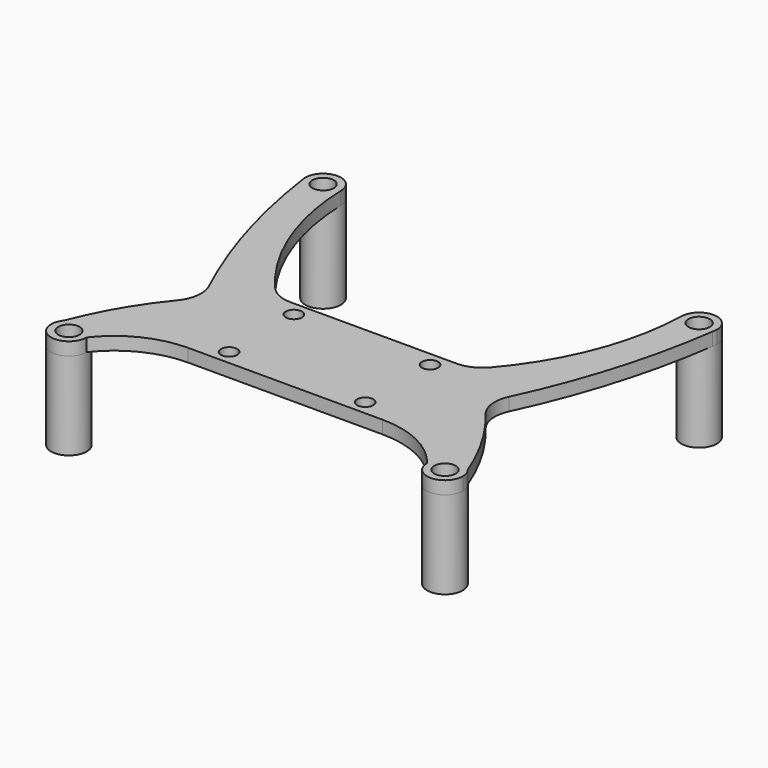
from build123d import *

# Parameters (mm, degrees)
F0_W     = 30
F0_H     = 17
F1_DEPTH = 2
F2_R     = 2.75
F3_DEPTH = 13.5
F4_R     = 5
F5_D     = 3.3
F5_DEPTH = 13.501
F6_D     = 3.3
F7_D     = 2.5


with BuildPart() as f1:
    # F0 (on Top) → F1 (new body)
    with BuildSketch(Plane.XY):
        with BuildLine():
            ThreePointArc((-31.125909, 1.744423), (-31.446933, 0.875424), (-31.75, 0))
            ThreePointArc((-31.75, 0), (-29, -2.75), (-26.25, 0))
            ThreePointArc((-26.25, 0), (-28.073649, 2.589281), (-31.125909, 1.744423))
        make_face()
        with BuildLine():
            ThreePointArc((-31.125909, 1.744423), (-31.589281, 0.926351), (-31.75, 0))
            ThreePointArc((-31.75, 0), (-31.446933, 0.875424), (-31.125909, 1.744423))
        make_face()
        with BuildLine():
            ThreePointArc((-31.125909, 1.744423), (-28.073649, 2.589281), (-26.25, 0))
            ThreePointArc((-26.25, 0), (-21.26124, 4.0514), (-15, 5.5))
            ThreePointArc((-15, 5.5), (-18.527929, 11.002842), (-21.688812, 16.724413))
            ThreePointArc((-21.688812, 16.724413), (-27.151344, 9.703113), (-31.125909, 1.744423))
        make_face()
        with Locations((0, 14)):
            Rectangle(F0_W, F0_H)
        with BuildLine():
            ThreePointArc((-21.688812, 16.724413), (-18.527929, 11.002842), (-15, 5.5))
            Line((-15, 5.5), (-15, 22.5))
            ThreePointArc((-15, 22.5), (-18.486529, 19.776801), (-21.688812, 16.724413))
        make_face()
        with BuildLine():
            ThreePointArc((-31.648811, 48.26088), (-27.981561, 32.078047), (-21.688812, 16.724413))
            ThreePointArc((-21.688812, 16.724413), (-18.486529, 19.776801), (-15, 22.5))
            ThreePointArc((-15, 22.5), (-23.091727, 34.702805), (-26.25, 49))
            ThreePointArc((-26.25, 49), (-28.626993, 46.275415), (-31.648811, 48.26088))
        make_face()
        with BuildLine():
            ThreePointArc((21.688812, 16.724413), (18.527929, 11.002842), (15, 5.5))
            ThreePointArc((15, 5.5), (21.26124, 4.0514), (26.25, 0))
            ThreePointArc((26.25, 0), (28.073649, 2.589281), (31.125909, 1.744423))
            ThreePointArc((31.125909, 1.744423), (27.151344, 9.703113), (21.688812, 16.724413))
        make_face()
        with BuildLine():
            Line((15, 22.5), (15, 5.5))
            ThreePointArc((15, 5.5), (18.527929, 11.002842), (21.688812, 16.724413))
            ThreePointArc((21.688812, 16.724413), (18.486529, 19.776801), (15, 22.5))
        make_face()
        with BuildLine():
            ThreePointArc((-31.75, 49), (-31.700095, 48.630345), (-31.648811, 48.26088))
            ThreePointArc((-31.648811, 48.26088), (-28.626993, 46.275415), (-26.25, 49))
            ThreePointArc((-26.25, 49), (-29, 51.75), (-31.75, 49))
        make_face()
        with BuildLine():
            ThreePointArc((-31.75, 49), (-31.724585, 48.626993), (-31.648811, 48.26088))
            ThreePointArc((-31.648811, 48.26088), (-31.700095, 48.630345), (-31.75, 49))
        make_face()
        with BuildLine():
            ThreePointArc((26.25, 49), (23.091727, 34.702805), (15, 22.5))
            ThreePointArc((15, 22.5), (18.486529, 19.776801), (21.688812, 16.724413))
            ThreePointArc((21.688812, 16.724413), (27.981561, 32.078047), (31.648811, 48.26088))
            ThreePointArc((31.648811, 48.26088), (28.626993, 46.275415), (26.25, 49))
        make_face()
        with BuildLine():
            ThreePointArc((31.125909, 1.744423), (28.073649, 2.589281), (26.25, 0))
            ThreePointArc((26.25, 0), (29, -2.75), (31.75, 0))
            ThreePointArc((31.75, 0), (31.446933, 0.875424), (31.125909, 1.744423))
        make_face()
        with BuildLine():
            ThreePointArc((31.75, 49), (29, 51.75), (26.25, 49))
            ThreePointArc((26.25, 49), (28.626993, 46.275415), (31.648811, 48.26088))
            ThreePointArc((31.648811, 48.26088), (31.700095, 48.630345), (31.75, 49))
        make_face()
        with BuildLine():
            ThreePointArc((31.125909, 1.744423), (31.446933, 0.875424), (31.75, 0))
            ThreePointArc((31.75, 0), (31.589281, 0.926351), (31.125909, 1.744423))
        make_face()
        with BuildLine():
            ThreePointArc((31.75, 49), (31.700095, 48.630345), (31.648811, 48.26088))
            ThreePointArc((31.648811, 48.26088), (31.724585, 48.626993), (31.75, 49))
        make_face()
    extrude(amount=F1_DEPTH)

    # F2 (on face) → F3 (join)
    with BuildSketch(Plane(origin=(0, 0, 0), x_dir=(1, 0, 0), z_dir=(0, 0, -1))):
        with Locations((29, 0)):
            Circle(F2_R)
        with Locations((-29, 0)):
            Circle(F2_R)
        with Locations((29, -49)):
            Circle(F2_R)
        with Locations((-29, -49)):
            Circle(F2_R)
    extrude(amount=F3_DEPTH)

    # F4
    f4_edges = [f1.edges().sort_by_distance(p)[0] for p in [
        (15, 22.5, 1),
        (-15, 22.5, 1),
        (-21.688812, 16.724413, 1),
        (21.688812, 16.724413, 1),
    ]]
    fillet(f4_edges, radius=F4_R)

    # F5 (through all, one way)
    with BuildSketch(Plane.XY):
        with Locations((29, 0), (-29, 0), (-29, 49), (29, 49)):
            Circle(F5_D / 2)
    extrude(amount=-F5_DEPTH, mode=Mode.SUBTRACT)

    # F6 (through all)
    with Locations(Plane(origin=(0, 0, 0), x_dir=(1, 0, 0), z_dir=(0, 0, -1))):
        with Locations((-29, 0), (29, 0), (-29, -49), (29, -49)):
            Hole(F6_D / 2)

    # F7 (through all)
    with Locations(Plane(origin=(0, 0, 0), x_dir=(1, 0, 0), z_dir=(0, 0, -1))):
        with Locations((-10.5, -7.75), (-10.5, -20.25), (10.5, -20.25), (10.5, -7.75)):
            Hole(F7_D / 2)


solid = f1.part
